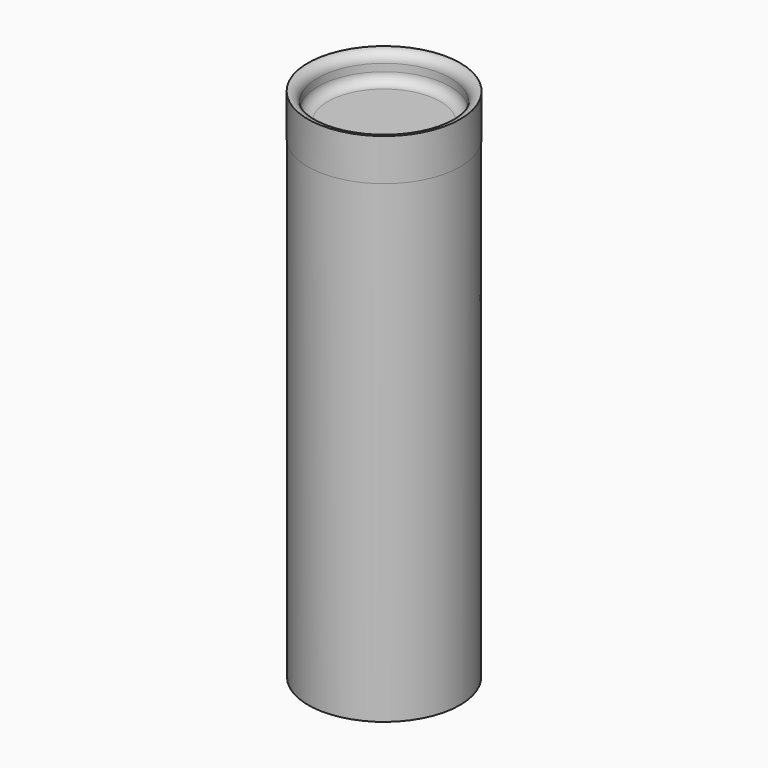
from build123d import *

# Parameters (mm, degrees)
F0_R     = 38.628552608
F0_R_2   = 35.5829437887
F1_DEPTH = 241.3
F2_R     = 38.7684611147
F3_DEPTH = 21.336
F4_R     = 33.724483213
F5_DEPTH = 13.97
F8_DEPTH = 59.944


# Not quite as in the source:
# - a fillet or chamfer that OpenCascade refuses, or shapes differently, is made with other operations: its cross-section is extruded or revolved along the edge and cut away or added


with BuildPart() as f1:
    # F0 (on Top) → F1 (new body)
    with BuildSketch(Plane.XY):
        Circle(F0_R)
        Circle(F0_R_2, mode=Mode.SUBTRACT)
    extrude(amount=F1_DEPTH)

    # F2 (on face) → F3 (join)
    with BuildSketch(Plane.XY.offset(241.3)):
        Circle(F2_R)
    extrude(amount=F3_DEPTH)

    # F4 (on face) → F5 (cut)
    with BuildSketch(Plane.XY.offset(262.636)):
        Circle(F4_R)
    extrude(amount=-F5_DEPTH, mode=Mode.SUBTRACT)

    # F6: fillet of radius 5.08 on 3 edges, made by hand

    # F6_s1 → F6_t2 (revolve)
    with BuildSketch(Plane.XZ):
        with BuildLine():
            ThreePointArc((33.724483213, 253.746), (32.2365856615, 250.1538975516), (28.644483213, 248.666))
            Line((28.644483213, 248.666), (33.724483213, 248.666))
            Line((33.724483213, 248.666), (33.724483213, 253.746))
        make_face()
    revolve(axis=Axis((0, 0, 248.666), (0, 0, 1)))

    # F6_s3 → F6_t4 (revolve, cut)
    with BuildSketch(Plane.XZ):
        with BuildLine():
            ThreePointArc((38.804483213, 262.636), (35.2123807646, 261.1481024484), (33.724483213, 257.556))
            Line((33.724483213, 257.556), (33.724483213, 262.636))
            Line((33.724483213, 262.636), (38.804483213, 262.636))
        make_face()
    revolve(axis=Axis((0, 0, 262.636), (0, 0, 1)), mode=Mode.SUBTRACT)

    # F7 (on Front) → F8 (cut)
    with BuildSketch(Plane.XZ):
        Polygon((-21.0285011722, 108.1128418446), (-33.6541458964, 177.6677370071), (-26.883315295, 104.4196635485), (0, 93.3401212096), (25.4367366433, 104.4196635485), (32.8230932355, 176.4366775751), (19.8969673365, 108.1128418446), (0, 99.4462705343), align=None)
    extrude(amount=-F8_DEPTH, mode=Mode.SUBTRACT)


solid = f1.part
